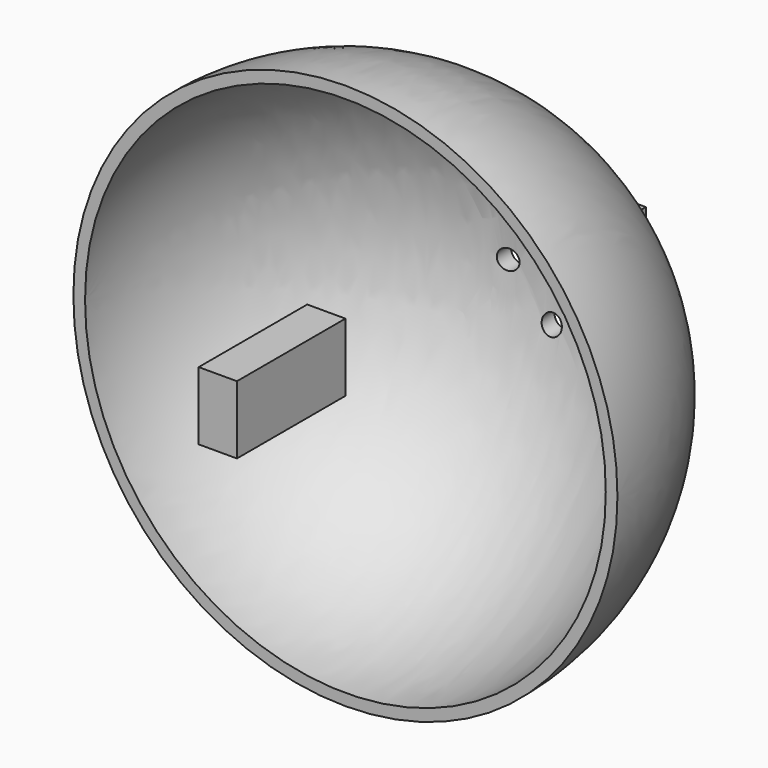
from build123d import *

# Parameters (mm, degrees)
F1_ANGLE = 180
F3_W     = 7.0469270903
F3_H     = 12.5417197123
F4_DEPTH = 25
F5_W     = 4.6478901516
F5_H     = 30
F6_DEPTH = 15
F7_ANGLE = 180
F8_R     = 1.85
F9_DEPTH = 60


# Not quite as in the source:
# - a feature names something its author has since deleted; it is built from what else it names


with BuildPart() as f1:
    # F0 (on Front) → F1 (revolve)
    with BuildSketch(Plane.XZ):
        with BuildLine():
            Line((0, 0), (100.295685879, 0))
            ThreePointArc((100.295685879, 0), (50.1478429395, 50.366821709), (0, 0))
        make_face()
    revolve(axis=Axis((50.1478429395, 0, 0), (-1, 0, 0)), revolution_arc=F1_ANGLE)

    # F5 (on face) → F6 (join, symmetric)
    with BuildSketch(Plane.YZ.offset(50.1478429395)):
        with Locations((48.1690146605, 0)):
            Rectangle(F5_W, F5_H)
    extrude(amount=F6_DEPTH, both=True)

    # F2 (on Front) → F7 (revolve, cut)
    with BuildSketch(Plane.XZ):
        with BuildLine():
            Line((2.1483402697, 0), (98.1473456093, 0))
            ThreePointArc((98.1473456093, 0), (50.1478429395, 48.2185027448), (2.1483402697, 0))
        make_face()
    revolve(axis=Axis((50.1478429395, 0, 0), (-1, 0, 0)), revolution_arc=F7_ANGLE, mode=Mode.SUBTRACT)

    # F8 (on Front) → F9 (cut)
    with BuildSketch(Plane.XZ):
        with BuildLine():
            ThreePointArc((51.9978429395, 8.2185027448), (48.8396953943, 9.52665029), (50.1478429395, 6.3685027448))
            ThreePointArc((50.1478429395, 6.3685027448), (51.4559904847, 6.9103551996), (51.9978429395, 8.2185027448))
        make_face()
        with Locations((42.1478429395, 0.2185027448)):
            Circle(F8_R)
        with BuildLine():
            ThreePointArc((59.9978429395, 0.2185027448), (58.1478429395, 2.0685027448), (56.2978429395, 0.2185027448))
            ThreePointArc((56.2978429395, 0.2185027448), (58.1478429395, -1.6314972552), (59.9978429395, 0.2185027448))
        make_face()
        with BuildLine():
            ThreePointArc((51.9978429395, -7.7814972552), (51.4559904847, -6.47334971), (50.1478429395, -5.9314972552))
            ThreePointArc((50.1478429395, -5.9314972552), (48.8396953943, -9.0896448004), (51.9978429395, -7.7814972552))
        make_face()
    extrude(amount=-F9_DEPTH, mode=Mode.SUBTRACT)


with BuildPart() as f4:
    # F3 (on Front) → F4 (new body)
    with BuildSketch(Plane.XZ):
        with Locations((46.6243793944, 6.2708598562)):
            Rectangle(F3_W, F3_H)
    extrude(amount=F4_DEPTH)


solid = Compound([f1.part, f4.part])
